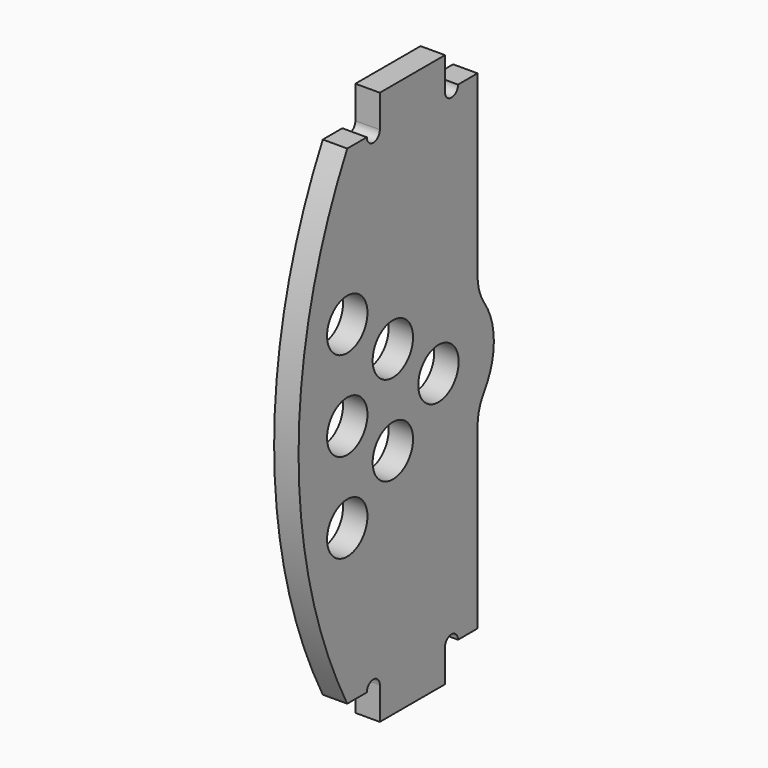
from build123d import *

# Parameters (mm, degrees)
F0_R     = 1.55
F1_DEPTH = 1.5
F2_W     = 5
F2_H     = 2
F3_DEPTH = 1.5
F4_R     = 0.5
F5_DEPTH = 25
F7_DEPTH = 1.5
F8_R     = 3


with BuildPart() as f1:
    # F0 (on Right) → F1 (new body)
    with BuildSketch(Plane.YZ):
        with BuildLine():
            Line((-10, 0), (0, 0))
            Line((0, 0), (0, 30))
            Line((0, 30), (-10, 30))
            ThreePointArc((-10, 30), (-13.7334119498, 15), (-10, 0))
        make_face()
        with Locations((-10, 9.5)):
            Circle(F0_R, mode=Mode.SUBTRACT)
        with Locations((-6.5, 12.25)):
            Circle(F0_R, mode=Mode.SUBTRACT)
        with Locations((-10, 15)):
            Circle(F0_R, mode=Mode.SUBTRACT)
        with Locations((-10, 20.5)):
            Circle(F0_R, mode=Mode.SUBTRACT)
        with Locations((-6.5, 17.75)):
            Circle(F0_R, mode=Mode.SUBTRACT)
        with Locations((-3, 15)):
            Circle(F0_R, mode=Mode.SUBTRACT)
    extrude(amount=F1_DEPTH)

    # F2 (on face) → F3 (join)
    with BuildSketch(Plane.YZ.offset(1.5)):
        with Locations((-5, 31)):
            Rectangle(F2_W, F2_H)
        with Locations((-5, -1)):
            Rectangle(F2_W, F2_H)
    extrude(amount=-F3_DEPTH)

    # F4 (on face) → F5 (cut)
    with BuildSketch(Plane.YZ.offset(1.5)):
        with Locations((-8, 30)):
            Circle(F4_R)
        with Locations((-2, 30)):
            Circle(F4_R)
        with Locations((-2, 0)):
            Circle(F4_R)
        with Locations((-8, 0)):
            Circle(F4_R)
    extrude(amount=-F5_DEPTH, mode=Mode.SUBTRACT)

    # F6 (on face) → F7 (join)
    with BuildSketch(Plane.YZ.offset(1.5)):
        with BuildLine():
            Line((0, 18.0103986447), (0, 11.9896013553))
            ThreePointArc((0, 11.9896013553), (1.25, 15), (0, 18.0103986447))
        make_face()
    extrude(amount=-F7_DEPTH)

    # F8
    f8_edges = [f1.edges().sort_by_distance(p)[0] for p in [
        (0.75, 0, 11.989601),
        (0.75, 0, 18.010399),
    ]]
    fillet(f8_edges, radius=F8_R)


solid = f1.part
